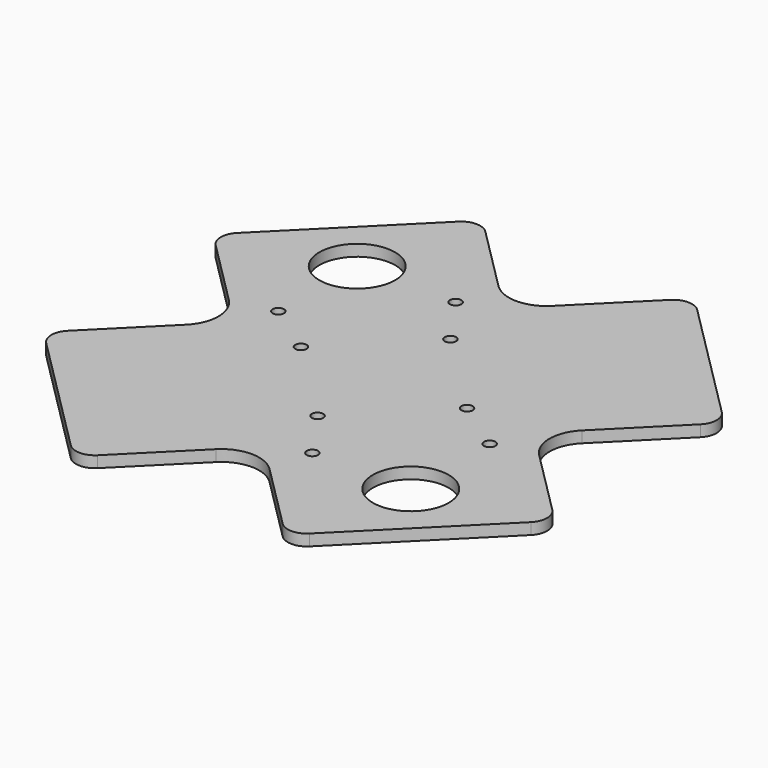
from build123d import *

# Parameters (mm, degrees)
F0_R     = 1.5
F0_R_2   = 10
F1_DEPTH = 3
F2_R     = 5


with BuildPart() as f1:
    # F0 (on Top) → F1 (new body)
    with BuildSketch(Plane.XY):
        with BuildLine():
            Line((67.5, 27.96), (27.96, 67.5))
            Line((27.96, 67.5), (7.0710678119, 46.6110678119))
            ThreePointArc((7.0710678119, 46.6110678119), (0, 43.6821356237), (-7.0710678119, 46.6110678119))
            Line((-7.0710678119, 46.6110678119), (-27.96, 67.5))
            Line((-27.96, 67.5), (-67.5, 27.96))
            Line((-67.5, 27.96), (-46.6110678119, 7.0710678119))
            ThreePointArc((-46.6110678119, 7.0710678119), (-43.6821356237, 0), (-46.6110678119, -7.0710678119))
            Line((-46.6110678119, -7.0710678119), (-67.5, -27.96))
            Line((-67.5, -27.96), (-27.96, -67.5))
            Line((-27.96, -67.5), (-7.0710678119, -46.6110678119))
            ThreePointArc((-7.0710678119, -46.6110678119), (0, -43.6821356237), (7.0710678119, -46.6110678119))
            Line((7.0710678119, -46.6110678119), (27.96, -67.5))
            Line((27.96, -67.5), (67.5, -27.96))
            Line((67.5, -27.96), (46.6110678119, -7.0710678119))
            ThreePointArc((46.6110678119, -7.0710678119), (43.6821356237, 0), (46.6110678119, 7.0710678119))
            Line((46.6110678119, 7.0710678119), (67.5, 27.96))
        make_face()
        with Locations((9.5, -35.5)):
            Circle(F0_R, mode=Mode.SUBTRACT)
        with Locations((35.3553390593, -35.3553390593)):
            Circle(F0_R_2, mode=Mode.SUBTRACT)
        with Locations((0, -21.9203102168)):
            Circle(F0_R, mode=Mode.SUBTRACT)
        with Locations((35.5, -9.5)):
            Circle(F0_R, mode=Mode.SUBTRACT)
        with Locations((-35.5, 9.5)):
            Circle(F0_R, mode=Mode.SUBTRACT)
        with Locations((-21.9203102168, 0)):
            Circle(F0_R, mode=Mode.SUBTRACT)
        with Locations((-35.3553390593, 35.3553390593)):
            Circle(F0_R_2, mode=Mode.SUBTRACT)
        with Locations((-9.5, 35.5)):
            Circle(F0_R, mode=Mode.SUBTRACT)
        with Locations((21.9203102168, 0)):
            Circle(F0_R, mode=Mode.SUBTRACT)
        with Locations((0, 21.9203102168)):
            Circle(F0_R, mode=Mode.SUBTRACT)
    extrude(amount=F1_DEPTH)

    # F2
    f2_edges = [f1.edges().sort_by_distance(p)[0] for p in [
        (27.96, -67.5, 1.5),
        (67.5, -27.96, 1.5),
        (67.5, 27.96, 1.5),
        (27.96, 67.5, 1.5),
        (-27.96, 67.5, 1.5),
        (-67.5, 27.96, 1.5),
        (-67.5, -27.96, 1.5),
        (-27.96, -67.5, 1.5),
    ]]
    fillet(f2_edges, radius=F2_R)


solid = f1.part
